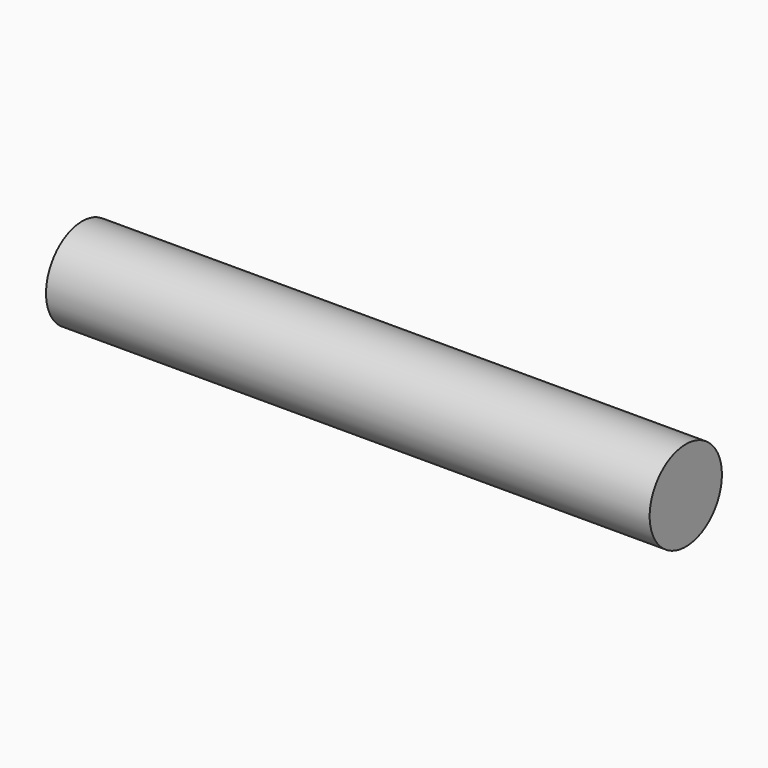
from build123d import *

# Parameters (mm, degrees)
F0_R     = 1.14
F1_DEPTH = 7.62


# Not quite as in the source:
# - the program builds the solid bodies; features that only make, move or delete a surface that nothing else refers to are left out


with BuildPart() as f1:
    # F0 (on Right) → F1 (new body, symmetric)
    with BuildSketch(Plane.YZ):
        Circle(F0_R)
    extrude(amount=F1_DEPTH, both=True)


solid = f1.part
